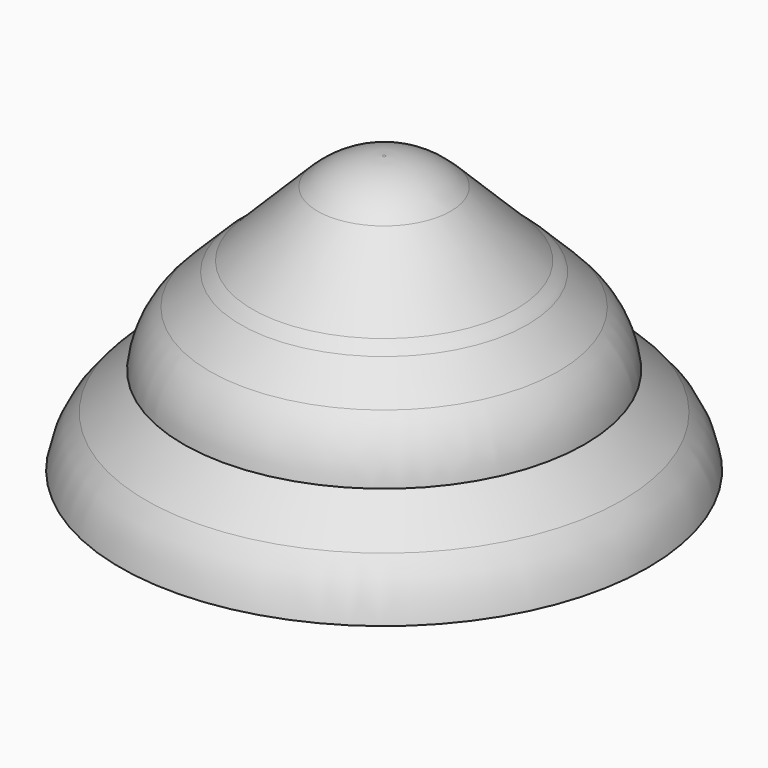
from build123d import *

# Parameters (mm, degrees)
F0_R        = 36.3127781595
F1_DEPTH    = 76.2
F0_R_2      = 55.3433829245
F2_DEPTH    = 50.8
F0_R_3      = 72.7478178249
F3_DEPTH    = 25.4
F4_SIZE     = 25.39999
F5_S5_R     = 55.3433829245
F5_T6_DEPTH = 105


# Not quite as in the source:
# - a fillet or chamfer that OpenCascade refuses, or shapes differently, is made with other operations: its cross-section is extruded or revolved along the edge and cut away or added
# - a fillet or chamfer is up to 0.001 mm smaller than in the source, because OpenCascade refuses the exact size


with BuildPart() as f1:
    # F0 (on Top) → F1 (new body)
    with BuildSketch(Plane.XY):
        Circle(F0_R)
    extrude(amount=F1_DEPTH)

    # F0 (on Top) → F2 (join)
    with BuildSketch(Plane.XY):
        Circle(F0_R_2)
        Circle(F0_R, mode=Mode.SUBTRACT)
    extrude(amount=F2_DEPTH)

    # F0 (on Top) → F3 (join)
    with BuildSketch(Plane.XY):
        Circle(F0_R_3)
        Circle(F0_R_2, mode=Mode.SUBTRACT)
    extrude(amount=F3_DEPTH)

    # F4 (size 25.4 in the source; OpenCascade refuses exactly that, so slightly less here)
    f4_edges = [f1.edges().sort_by_distance(p)[0] for p in [
        (-36.312778, 0, 76.2),
    ]]
    chamfer(f4_edges, length=F4_SIZE)

    # F5: chamfer of 18.542 on 2 edges, made by hand


with BuildPart() as f5_tool2:
    # F5_s3 → F5_t4 (revolve)
    with BuildSketch(Plane.XZ):
        Polygon((54.2058178249, 25.4), (72.7478178249, 6.858), (72.7478178249, 25.4), align=None)
    revolve(axis=Axis((0, 0, 25.4), (0, 0, 1)))

    # F5_s5 → F5_t6 (cut, symmetric)
    with BuildSketch(Plane.XY.offset(16.1)):
        Circle(F5_S5_R)
    extrude(amount=F5_T6_DEPTH, both=True, mode=Mode.SUBTRACT)


with BuildPart() as f1_1:
    add(f1.part)

    # F5_t1: cut F5_tool2
    add(f5_tool2.part, mode=Mode.SUBTRACT)

    # F5_s7 → F5_t8 (revolve, cut)
    with BuildSketch(Plane.XZ):
        Polygon((36.8013829245, 50.8), (55.3433829245, 32.258), (55.3433829245, 50.8), align=None)
    revolve(axis=Axis((0, 0, 50.8), (0, 0, 1)), mode=Mode.SUBTRACT)

    # F6: fillet of radius 25.4 on 4 edges, made by hand

    # F6_s1 → F6_t2 (revolve, cut)
    with BuildSketch(Plane.XZ):
        with BuildLine():
            ThreePointArc((18.3522759174, 68.7605122421), (10.1119228573, 74.2665401258), (0.3917636752, 76.2))
            Line((0.3917636752, 76.2), (0.3917636752, 76.708))
            Line((0.3917636752, 76.708), (11.1232086492, 76.708))
            Line((11.1232086492, 76.708), (18.7114861622, 69.119722487))
            Line((18.7114861622, 69.119722487), (18.3522759174, 68.7605122421))
        make_face()
    revolve(axis=Axis((0, 0, 76.2), (0, 0, 1)), mode=Mode.SUBTRACT)

    # F6_s3 → F6_t4 (revolve, cut)
    with BuildSketch(Plane.XZ):
        with BuildLine():
            ThreePointArc((48.0441667783, 39.5572161462), (53.0070025329, 32.5365446991), (55.3433829245, 24.2624349004))
            Line((55.3433829245, 24.2624349004), (55.8485774923, 24.3157495203))
            ThreePointArc((55.8485774923, 24.3157495203), (55.8513829245, 28.2602174502), (55.8513829245, 32.258))
            Line((55.8513829245, 32.258), (55.7025931693, 32.6172102448))
            Line((55.7025931693, 32.6172102448), (48.4033770231, 39.9164263911))
            Line((48.4033770231, 39.9164263911), (48.0441667783, 39.5572161462))
        make_face()
    revolve(axis=Axis((0, 0, 32.258), (0, 0, 1)), mode=Mode.SUBTRACT)

    # F6_s5 → F6_t6 (revolve, cut)
    with BuildSketch(Plane.XZ):
        with BuildLine():
            ThreePointArc((65.6214802199, 13.984337605), (70.2919041112, 7.5564195951), (72.7478178249, 0))
            Line((72.7478178249, 0), (73.2495548219, 0.0795234927))
            ThreePointArc((73.2495548219, 0.0795234927), (73.2558178249, 3.429), (73.2558178249, 6.858))
            Line((73.2558178249, 6.858), (73.1070280697, 7.2172102448))
            Line((73.1070280697, 7.2172102448), (65.9806904647, 14.3435478499))
            Line((65.9806904647, 14.3435478499), (65.6214802199, 13.984337605))
        make_face()
    revolve(axis=Axis((0, 0, 6.858), (0, 0, 1)), mode=Mode.SUBTRACT)

    # F6_s7 → F6_t8 (revolve, cut)
    with BuildSketch(Plane.XZ):
        with BuildLine():
            ThreePointArc((36.3127781595, 50.8), (37.9669911758, 49.5120321576), (39.5093522451, 48.0920306794))
            Line((39.5093522451, 48.0920306794), (39.86856249, 48.4512409242))
            Line((39.86856249, 48.4512409242), (37.1605931693, 51.1592102448))
            Line((37.1605931693, 51.1592102448), (36.8013829245, 51.308))
            ThreePointArc((36.8013829245, 51.308), (36.557080542, 51.308), (36.6080569226, 51.2133696313))
            Line((36.6080569226, 51.2133696313), (36.3127781595, 50.8))
        make_face()
    revolve(axis=Axis((0, 0, 50.8), (0, 0, 1)), mode=Mode.SUBTRACT)


solid = f1_1.part
